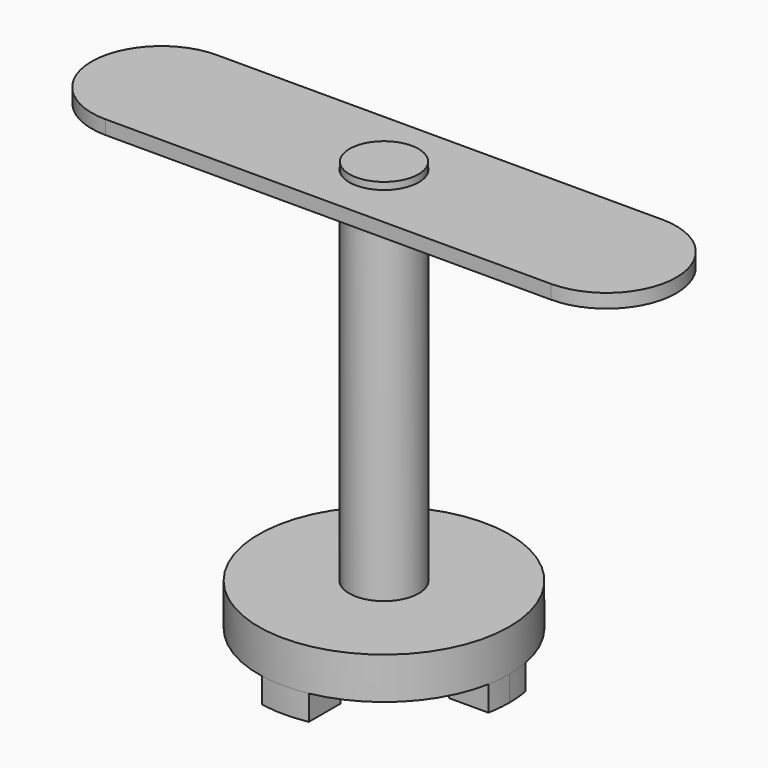
from build123d import *

# Parameters (mm, degrees)
F0_R     = 2.5
F1_DEPTH = 25
F0_R_2   = 9
F0_R_3   = 5
F2_DEPTH = 3
F3_R     = 2.475
F4_DEPTH = 1.8
F5_R     = 2.475
F6_DEPTH = 1.5
F5_R_2   = 4
F5_R_3   = 2.5
F7_DEPTH = 1


# Not quite as in the source:
# - after a boolean that leaves OpenCascade's solid faulty, fix() repairs it


with BuildPart() as f1:
    # F0 (on Top) → F1 (new body)
    with BuildSketch(Plane.XY):
        Circle(F0_R)
    extrude(amount=F1_DEPTH)

    # F0 (on Top) → F2 (join)
    with BuildSketch(Plane.XY):
        Circle(F0_R_2)
        Circle(F0_R_3, mode=Mode.SUBTRACT)
        Circle(F0_R_3)
        Circle(F0_R, mode=Mode.SUBTRACT)
        Circle(F0_R)
    extrude(amount=-F2_DEPTH)

    # F3 (on face) → F4 (join)
    with BuildSketch(Plane(origin=(0, 0, -3), x_dir=(1, 0, 0), z_dir=(0, 0, -1))):
        Circle(F3_R)
        with BuildLine():
            Line((-6.0041221744, 1.6499974638), (-8.8474577348, 1.6499974638))
            ThreePointArc((-8.8474577348, 1.6499974638), (-8.9999640282, -0.0254458428), (-8.837986196, -1.7))
            Line((-8.837986196, -1.7), (-6, -1.7))
            Line((-6, -1.7), (-6.0041221744, 1.6499974638))
        make_face()
        with BuildLine():
            Line((-1.675, 8.8427583366), (-1.675, 6))
            Line((-1.675, 6), (1.6749974638, 6.0041221744))
            Line((1.6749974638, 6.0041221744), (1.6749974638, 8.842758817))
            ThreePointArc((1.6749974638, 8.842758817), (-1.2906e-06, 9), (-1.675, 8.8427583366))
        make_face()
        with BuildLine():
            ThreePointArc((9, 0), (8.9606033566, 0.841182195), (8.8427583366, 1.675))
            Line((8.8427583366, 1.675), (6.025, 1.675))
            Line((6.025, 1.675), (6.0291221744, -1.6749974638))
            Line((6.0291221744, -1.6749974638), (8.842758817, -1.6749974638))
            ThreePointArc((8.842758817, -1.6749974638), (8.9606034773, -0.84118091), (9, 0))
        make_face()
        with BuildLine():
            Line((-1.6499974638, -6.0291221744), (-1.6499974638, -8.8474577348))
            ThreePointArc((-1.6499974638, -8.8474577348), (0.0254458428, -8.9999640282), (1.7, -8.837986196))
            Line((1.7, -8.837986196), (1.7, -6.025))
            Line((1.7, -6.025), (-1.6499974638, -6.0291221744))
        make_face()
    extrude(amount=F4_DEPTH)

    add(f1.part.fix(), mode=Mode.REPLACE)

    # F5 (on face) → F6 (join)
    with BuildSketch(Plane.XY.offset(25)):
        Circle(F5_R)
    extrude(amount=F6_DEPTH)


with BuildPart() as f7:
    # F5 (on face) → F7 (new body)
    with BuildSketch(Plane.XY.offset(25)):
        with BuildLine():
            Line((16, 5), (-16, 5))
            ThreePointArc((-16, 5), (-21, 0), (-16, -5))
            Line((-16, -5), (16, -5))
            ThreePointArc((16, -5), (21, 0), (16, 5))
        make_face()
        Circle(F5_R_2, mode=Mode.SUBTRACT)
        Circle(F5_R_2)
        Circle(F5_R_3, mode=Mode.SUBTRACT)
    extrude(amount=F7_DEPTH)


solid = Compound([f1.part, f7.part])
